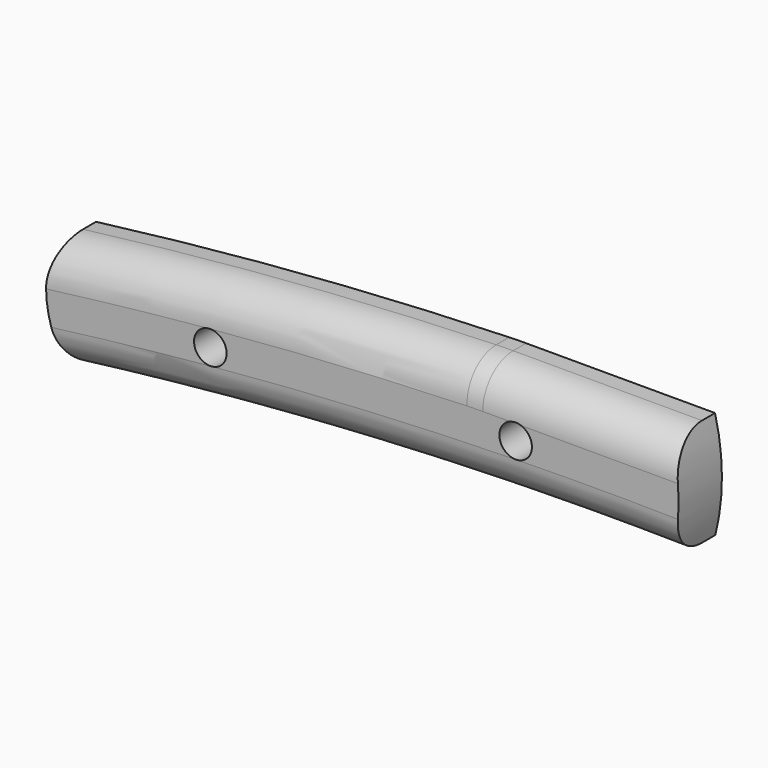
from build123d import *

# Parameters (mm, degrees)
F0_R        = 3
F1_DEPTH    = 10
F2_T1_DEPTH = 52.3011751173
F2_T4_ANGLE = 6.7239804363
F2_T6_ANGLE = 10.729424982
F2_T8_ANGLE = 1.7828949869


# Not quite as in the source:
# - a fillet or chamfer that OpenCascade refuses, or shapes differently, is made with other operations: its cross-section is extruded or revolved along the edge and cut away or added


with BuildPart() as f1:
    # F0 (on Front) → F1 (new body)
    with BuildSketch(Plane.XZ):
        with BuildLine():
            ThreePointArc((16.7161625637, 9.1005522793), (15.1603559483, 9.0884488757), (13.604925944, 9.0521415948))
            ThreePointArc((13.604925944, 9.0521415948), (-24.5259537531, 6.9533029462), (-62.5132279063, 3.0371680453))
            ThreePointArc((-62.5132279063, 3.0371680453), (-63.4446975244, -7.2627028514), (-59.2295458713, -16.7066147888))
            ThreePointArc((-59.2295458713, -16.7066147888), (-3.9332598443, -11.7153648591), (51.5779973344, -10.6703047235))
            ThreePointArc((51.5779973344, -10.6703047235), (52.7884384629, -0.7810693697), (51.517337681, 9.1005522793))
            Line((51.517337681, 9.1005522793), (16.7161625637, 9.1005522793))
        make_face()
        with Locations((-33.4603461426, -3.8443253384)):
            Circle(F0_R, mode=Mode.SUBTRACT)
        with Locations((22.7880547631, -0.7167291473)):
            Circle(F0_R, mode=Mode.SUBTRACT)
    extrude(amount=F1_DEPTH)

    # F2: fillet of radius 7 on 4 edges, made by hand

    # F2_s2 → F2_t1 (cut)
    with BuildSketch(Plane.YZ.offset(16.7161625637)):
        with BuildLine():
            ThreePointArc((-3, 9.1005522793), (-7.9497474683, 7.0502997476), (-10, 2.1005522793))
            Line((-10, 2.1005522793), (-10, 9.1005522793))
            Line((-10, 9.1005522793), (-3, 9.1005522793))
        make_face()
    extrude(amount=F2_T1_DEPTH, mode=Mode.SUBTRACT)

    # F2_s3 → F2_t4 (revolve, cut)
    with BuildSketch(Plane(origin=(13.8732538603, 0, 0.4318388106), x_dir=(0, 1, 0), z_dir=(0.9995158932, 0, 0.0311123662))):
        with BuildLine():
            ThreePointArc((-3, 8.624477953), (-7.9497474683, 6.5742254213), (-10, 1.624477953))
            Line((-10, 1.624477953), (-10, 8.624477953))
            Line((-10, 8.624477953), (-3, 8.624477953))
        make_face()
    revolve(axis=Axis((38.4948189015, -10, -790.5605729296), (0, -1, 0)), revolution_arc=F2_T4_ANGLE, mode=Mode.SUBTRACT)

    # F2_s5 → F2_t6 (revolve, cut)
    with BuildSketch(Plane(origin=(-77.6853434409, 0, -11.5863862591), x_dir=(0, 1, 0), z_dir=(-0.9890600521, 0, -0.1475134342))):
        with BuildLine():
            ThreePointArc((-3, 7.5903844134), (-7.9497474683, 5.5401318817), (-10, 0.5903844134))
            Line((-10, 0.5903844134), (-10, 7.5903844134))
            Line((-10, 7.5903844134), (-3, 7.5903844134))
        make_face()
    revolve(axis=Axis((38.4948189015, -10, -790.5605729293), (0, 1, 0)), revolution_arc=F2_T6_ANGLE, mode=Mode.SUBTRACT)

    # F2_s7 → F2_t8 (revolve, cut)
    with BuildSketch(Plane.YZ.offset(16.7161625637)):
        with BuildLine():
            ThreePointArc((-3, 9.1005522793), (-7.9497474683, 7.0502997476), (-10, 2.1005522793))
            Line((-10, 2.1005522793), (-10, 9.1005522793))
            Line((-10, 9.1005522793), (-3, 9.1005522793))
        make_face()
    revolve(axis=Axis((16.7161625637, -10, -90.8994477206), (0, -1, 0)), revolution_arc=F2_T8_ANGLE, mode=Mode.SUBTRACT)


solid = f1.part
